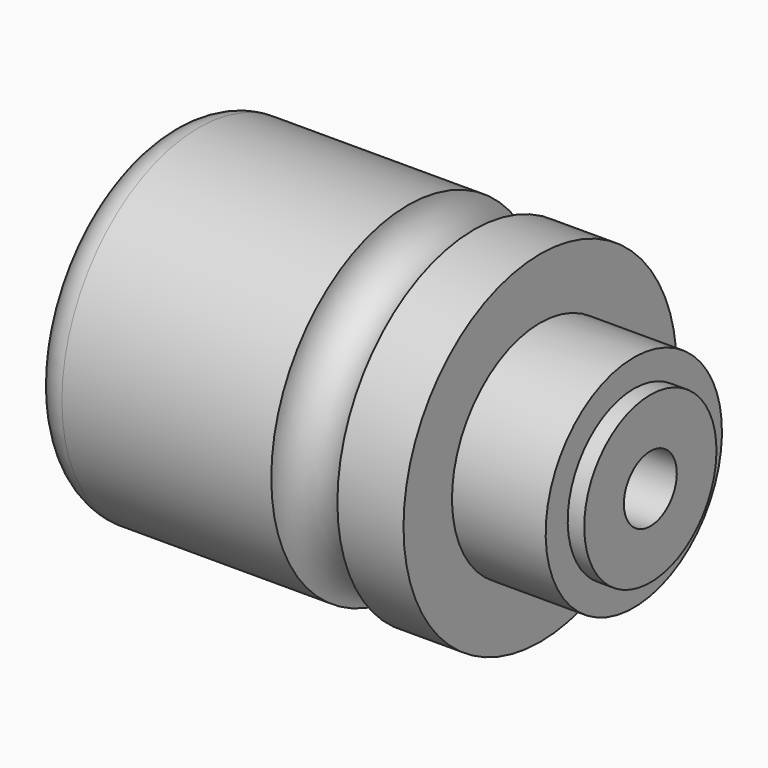
from build123d import *

# Parameters (mm, degrees)
F4_R = 5.99999


# Not quite as in the source:
# - a fillet or chamfer is up to 0.001 mm smaller than in the source, because OpenCascade refuses the exact size


with BuildPart() as f1:
    # F0 (on Front) → F1 (revolve)
    with BuildSketch(Plane.XZ):
        with BuildLine():
            Line((0, 31), (0, 0))
            Line((0, 0), (88, 0))
            Line((88, 0), (88, 15))
            Line((88, 15), (85, 15))
            Line((85, 15), (85, 20))
            Line((85, 20), (68, 20))
            Line((68, 20), (68, 31))
            Line((68, 31), (56, 31))
            ThreePointArc((56, 31), (50, 25), (44, 31))
            Line((44, 31), (0, 31))
        make_face()
    revolve(axis=Axis((44, 0, 0), (-1, 0, 0)))

    # F2 (on Front) → F3 (revolve, cut)
    with BuildSketch(Plane.XZ):
        Polygon((1.5, 25), (0, 25), (0, 0), (88, 0), (88, 6), (30, 6), (30, 16), (22, 16), (22, 20.5), (15, 20.5), (15, 12.5), (12, 12.5), (12, 16), (1.5, 16), align=None)
    revolve(axis=Axis((-11.4788431415, 0, 0), (-1, 0, 0)), mode=Mode.SUBTRACT)

    # F4 (radius 6 in the source; OpenCascade refuses exactly that, so slightly less here)
    f4_edges = [f1.edges().sort_by_distance(p)[0] for p in [
        (0, 0, -31),
    ]]
    fillet(f4_edges, radius=F4_R)


solid = f1.part
